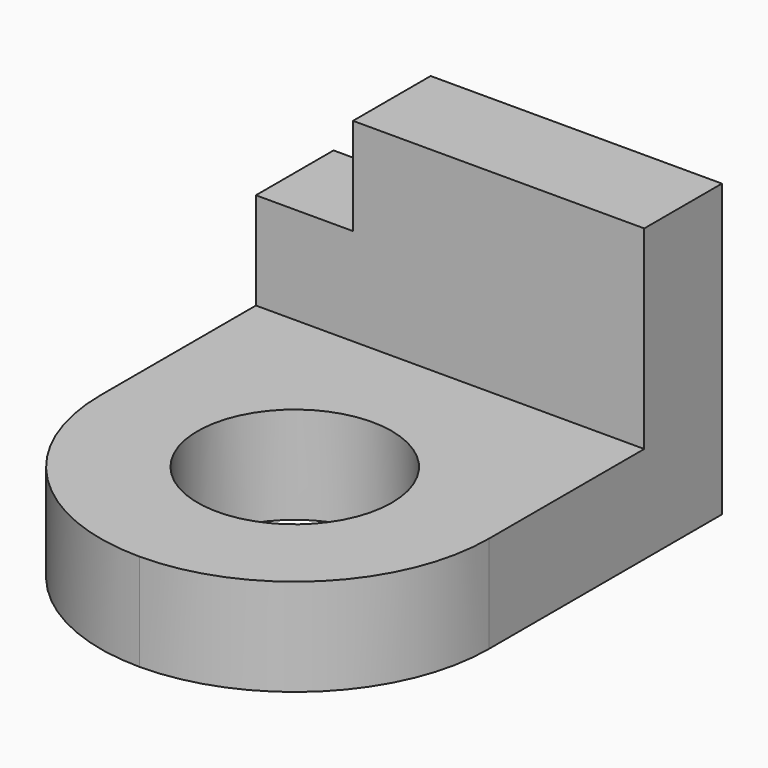
from build123d import *

# Parameters (mm, degrees)
F0_W     = 38.1
F0_H     = 12.7
F1_DEPTH = 12.7
F2_W     = 50.8
F2_H     = 12.7
F3_DEPTH = 50.8
F4_R     = 12.7
F5_DEPTH = 12.701
F6_R     = 25.39999


# Not quite as in the source:
# - a fillet or chamfer is up to 0.001 mm smaller than in the source, because OpenCascade refuses the exact size


with BuildPart() as f1:
    # F0 (on Front) → F1 (new body)
    with BuildSketch(Plane.XZ):
        Polygon((-25.4, 25.4), (-25.4, 0), (25.4, 0), (25.4, 25.4), (-12.7, 25.4), align=None)
        with Locations((6.35, 31.75)):
            Rectangle(F0_W, F0_H)
    extrude(amount=-F1_DEPTH)

    # F2 (on face) → F3 (join)
    with BuildSketch(Plane.XZ):
        with Locations((0, 6.35)):
            Rectangle(F2_W, F2_H)
    extrude(amount=F3_DEPTH)

    # F4 (on face) → F5 (cut, through all)
    with BuildSketch(Plane.XY.offset(12.7)):
        with Locations((0, -25.4)):
            Circle(F4_R)
    extrude(amount=-F5_DEPTH, mode=Mode.SUBTRACT)

    # F6 (radius 25.4 in the source; OpenCascade refuses exactly that, so slightly less here)
    f6_edges = [f1.edges().sort_by_distance(p)[0] for p in [
        (-25.4, -50.8, 6.35),
        (25.4, -50.8, 6.35),
    ]]
    fillet(f6_edges, radius=F6_R)


solid = f1.part
